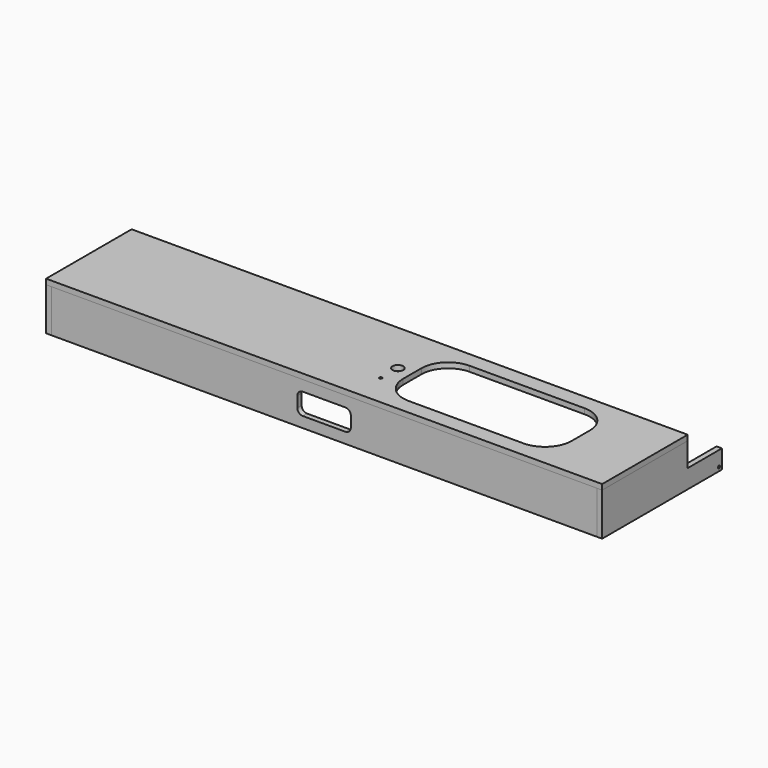
from build123d import *

# Parameters (mm, degrees)
F0_W      = 1320.8
F0_H      = 254
F1_DEPTH  = 12.7
F4_DEPTH  = 12.7
F5_D      = 6.35
F8_DEPTH  = 114.301
F9_R      = 12.7
F9_R_2    = 3.175
F10_DEPTH = 114.301
F12_W     = 1295.4
F12_H     = 101.6
F13_DEPTH = 12.7


with BuildPart() as f1:
    # F0 (on Top) → F1 (new body)
    with BuildSketch(Plane.XY):
        Rectangle(F0_W, F0_H)
    extrude(amount=-F1_DEPTH)

    # F7 (on Top) → F8 (cut, through all)
    with BuildSketch(Plane.XY):
        with BuildLine():
            ThreePointArc((508, 26.9875), (489.4012806053, 71.8887806053), (444.5, 90.4875))
            Line((444.5, 90.4875), (171.45, 90.4875))
            ThreePointArc((171.45, 90.4875), (126.5487193947, 71.8887806053), (107.95, 26.9875))
            Line((107.95, 26.9875), (107.95, -26.9875))
            ThreePointArc((107.95, -26.9875), (126.5487193947, -71.8887806053), (171.45, -90.4875))
            Line((171.45, -90.4875), (444.5, -90.4875))
            ThreePointArc((444.5, -90.4875), (489.4012806053, -71.8887806053), (508, -26.9875))
            Line((508, -26.9875), (508, 26.9875))
        make_face()
    extrude(amount=-F8_DEPTH, mode=Mode.SUBTRACT)

    # F9 (on Top) → F10 (cut, through all)
    with BuildSketch(Plane.XY):
        with Locations((73.66, 0)):
            Circle(F9_R)
        with Locations((73.406, -50.8)):
            Circle(F9_R_2)
    extrude(amount=-F10_DEPTH, mode=Mode.SUBTRACT)


with BuildPart() as f4:
    # F3 (on offset) → F4 (new body)
    with BuildSketch(Plane.YZ.offset(660.4)):
        Polygon((-127, -12.7), (-127, -114.3), (228.6, -114.3), (228.6, -69.85), (127, -69.85), (127, -12.7), (0, -12.7), align=None)
    extrude(amount=-F4_DEPTH)

    # F5 (through all)
    with Locations(Plane.YZ.offset(660.4)):
        with Locations((219.71, -105.41)):
            Hole(F5_D / 2)


with BuildPart() as f6_1:
    # F6: instance of F4
    add(f4.part.mirror(Plane.YZ))


with BuildPart() as f13:
    # F12 (on offset) → F13 (new body)
    with BuildSketch(Plane.XZ.offset(127)):
        with Locations((0, -63.5)):
            Rectangle(F12_W, F12_H)
        with BuildLine():
            ThreePointArc((63.5, -76.2), (59.7802561211, -85.1802561211), (50.8, -88.9))
            Line((50.8, -88.9), (-50.8, -88.9))
            ThreePointArc((-50.8, -88.9), (-59.7802561211, -85.1802561211), (-63.5, -76.2))
            Line((-63.5, -76.2), (-63.5, -50.8))
            ThreePointArc((-63.5, -50.8), (-59.7802561211, -41.8197438789), (-50.8, -38.1))
            Line((-50.8, -38.1), (50.8, -38.1))
            ThreePointArc((50.8, -38.1), (59.7802561211, -41.8197438789), (63.5, -50.8))
            Line((63.5, -50.8), (63.5, -76.2))
        make_face(mode=Mode.SUBTRACT)
    extrude(amount=-F13_DEPTH)


solid = Compound([f1.part, f4.part, f6_1.part, f13.part])
